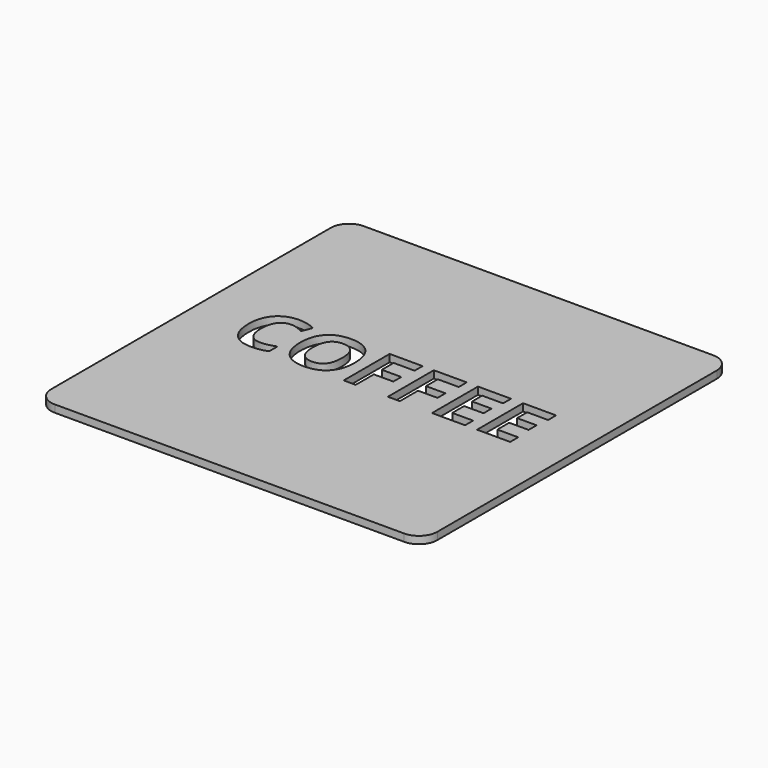
from build123d import *

# Parameters (mm, degrees)
F1_DEPTH     = 2
F2_TEXT_SIZE = 21.8775370679
F3_DEPTH     = 30


# Not quite as in the source:
# - Text() gives the source's letters only with a copy of the font that has no kerning and outlines rounded to 1/6400 em; it was checked with that copy


with BuildPart() as f1:
    # F0 (on Top) → F1 (new body)
    with BuildSketch(Plane.XY):
        with BuildLine():
            Line((-47.5, -52.5), (47.5, -52.5))
            ThreePointArc((47.5, -52.5), (51.0355339059, -51.0355339059), (52.5, -47.5))
            Line((52.5, -47.5), (52.5, 47.5))
            ThreePointArc((52.5, 47.5), (51.0355339059, 51.0355339059), (47.5, 52.5))
            Line((47.5, 52.5), (-47.5, 52.5))
            ThreePointArc((-47.5, 52.5), (-51.0355339059, 51.0355339059), (-52.5, 47.5))
            Line((-52.5, 47.5), (-52.5, -47.5))
            ThreePointArc((-52.5, -47.5), (-51.0355339059, -51.0355339059), (-47.5, -52.5))
        make_face()
    extrude(amount=F1_DEPTH)

    # F2 (on face) → F3 (cut)
    with BuildSketch(Plane.XY.offset(2)):
        with Locations((-39.8262285929, -5.561829306)):
            Text('COFFEE', F2_TEXT_SIZE, font='Open Sans', font_style=FontStyle.BOLD, text_align=(TextAlign.LEFT, TextAlign.BOTTOM))
    extrude(amount=-F3_DEPTH, mode=Mode.SUBTRACT)


solid = f1.part
